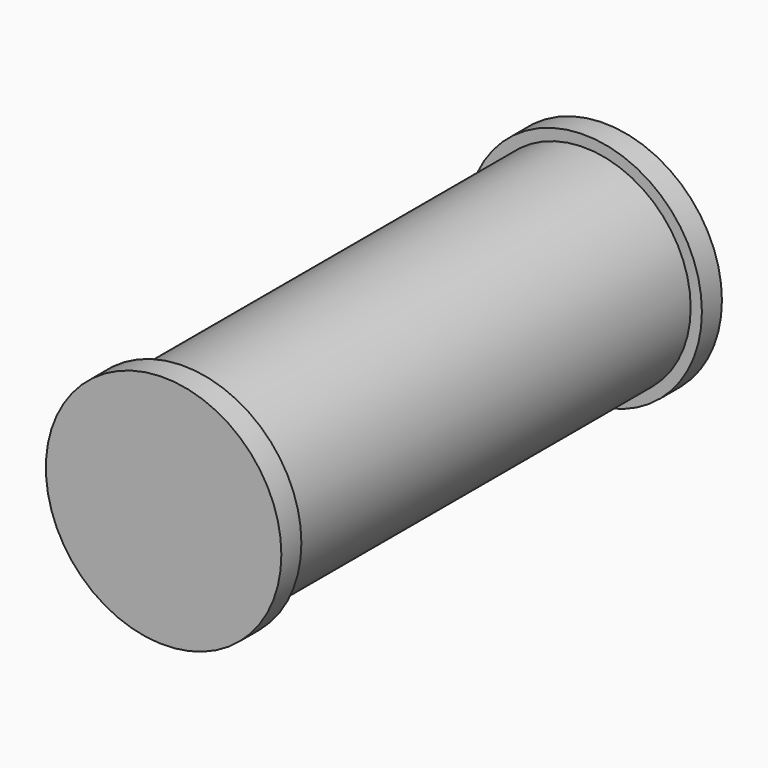
from build123d import *

# Parameters (mm, degrees)
F0_R          = 1.0812294985
F1_DEPTH      = 2.54
F1_DEPTH_BACK = 2.54
F2_R          = 1.1948962621
F3_DEPTH      = 0.254


# Not quite as in the source:
# - a pattern or mirror of a feature is missing from the dataset's text; its kind, count and spacing are read off the source's solid


with BuildPart() as f1:
    # F0 (on Front) → F1 (new body, two sides)
    with BuildSketch(Plane.XZ) as f1_sk:
        Circle(F0_R)
    extrude(amount=F1_DEPTH)
    extrude(f1_sk.sketch, amount=-F1_DEPTH_BACK)

    # F2 (on face) → F3 (join)
    with BuildSketch(Plane.XZ.offset(2.54)):
        Circle(F2_R)
    f3 = extrude(amount=F3_DEPTH)

    # F3_copies: F3 across plane
    add(f3.mirror(Plane.ZX))


solid = f1.part
